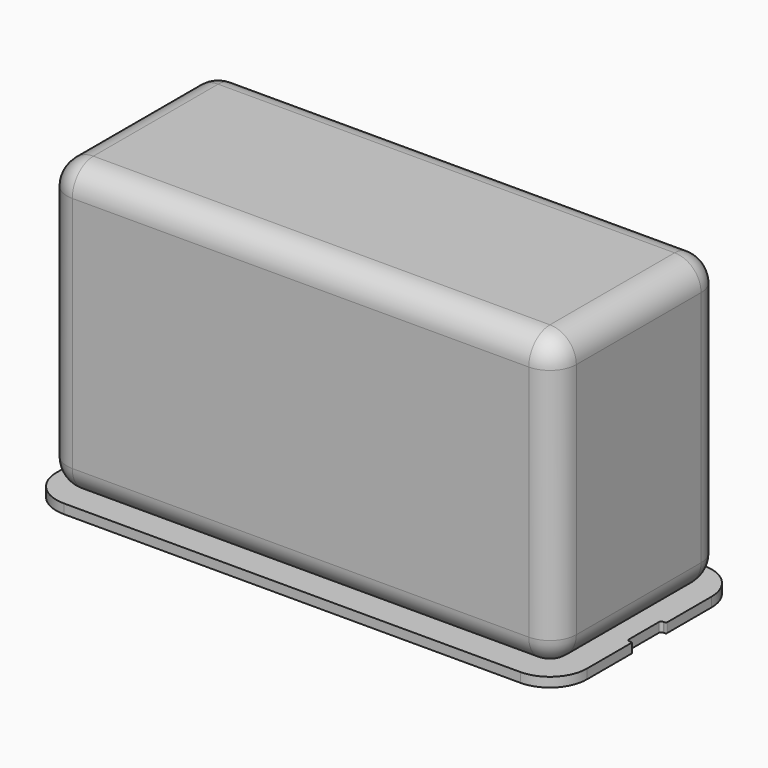
from build123d import *

# Parameters (mm, degrees)
F0_W      = 1004
F0_H      = 435
F1_DEPTH  = 18
F2_R      = 70
F3_W      = 70
F3_H      = 70
F4_DEPTH  = 2
F5_R      = 5
F6_W      = 20
F6_H      = 80
F7_DEPTH  = 18
F8_R      = 5
F9_W      = 964
F9_H      = 395
F10_DEPTH = 550
F11_R     = 50
F12_R     = 2


with BuildPart() as f1:
    # F0 (on Top) → F1 (new body)
    with BuildSketch(Plane.XY):
        Rectangle(F0_W, F0_H)
    extrude(amount=F1_DEPTH)

    # F2
    f2_edges = [f1.edges().sort_by_distance(p)[0] for p in [
        (-502, -217.5, 9),
        (-502, 217.5, 9),
        (502, 217.5, 9),
        (502, -217.5, 9),
    ]]
    fillet(f2_edges, radius=F2_R)

    # F3 (on face) → F4 (cut)
    with BuildSketch(Plane(origin=(0, 0, 0), x_dir=(1, 0, 0), z_dir=(0, 0, -1))):
        with Locations((-427, 142.5)):
            Rectangle(F3_W, F3_H)
        with Locations((-427, -142.5)):
            Rectangle(F3_W, F3_H)
        with Locations((427, -142.5)):
            Rectangle(F3_W, F3_H)
        with Locations((427, 142.5)):
            Rectangle(F3_W, F3_H)
    extrude(amount=-F4_DEPTH, mode=Mode.SUBTRACT)

    # F5
    f5_edges = [f1.edges().sort_by_distance(p)[0] for p in [
        (-462, -177.5, 1),
        (-392, -177.5, 1),
        (-462, -107.5, 1),
        (-392, -107.5, 1),
        (-392, 177.5, 1),
        (-462, 177.5, 1),
        (-392, 107.5, 1),
        (-462, 107.5, 1),
        (392, 107.5, 1),
        (462, 107.5, 1),
        (392, 177.5, 1),
        (462, 177.5, 1),
        (462, -107.5, 1),
        (392, -107.5, 1),
        (462, -177.5, 1),
        (392, -177.5, 1),
    ]]
    fillet(f5_edges, radius=F5_R)

    # F6 (on face) → F7 (cut)
    with BuildSketch(Plane.XY.offset(18)):
        with Locations((-502, 0)):
            Rectangle(F6_W, F6_H)
        with Locations((502, 0)):
            Rectangle(F6_W, F6_H)
    extrude(amount=-F7_DEPTH, mode=Mode.SUBTRACT)

    # F8
    f8_edges = [f1.edges().sort_by_distance(p)[0] for p in [
        (-492, 40, 9),
        (-492, -40, 9),
        (492, -40, 9),
        (492, 40, 9),
    ]]
    fillet(f8_edges, radius=F8_R)

    # F12
    f12_edges = [f1.edges().sort_by_distance(p)[0] for p in [
        (-502, -40, 9),
        (-502, 40, 9),
        (502, 40, 9),
        (502, -40, 9),
    ]]
    fillet(f12_edges, radius=F12_R)


with BuildPart() as f10:
    # F9 (on face) → F10 (new body)
    with BuildSketch(Plane.XY.offset(18)):
        Rectangle(F9_W, F9_H)
    extrude(amount=F10_DEPTH)

    # F11
    f11_edges = [f10.edges().sort_by_distance(p)[0] for p in [
        (482, 0, 568),
        (-482, 0, 568),
        (0, -197.5, 568),
        (482, -197.5, 293),
        (-482, -197.5, 293),
        (0, -197.5, 18),
        (482, 0, 18),
        (482, 197.5, 293),
        (0, 197.5, 568),
        (0, 197.5, 18),
        (-482, 197.5, 293),
        (-482, 0, 18),
    ]]
    fillet(f11_edges, radius=F11_R)


solid = Compound([f1.part, f10.part])
